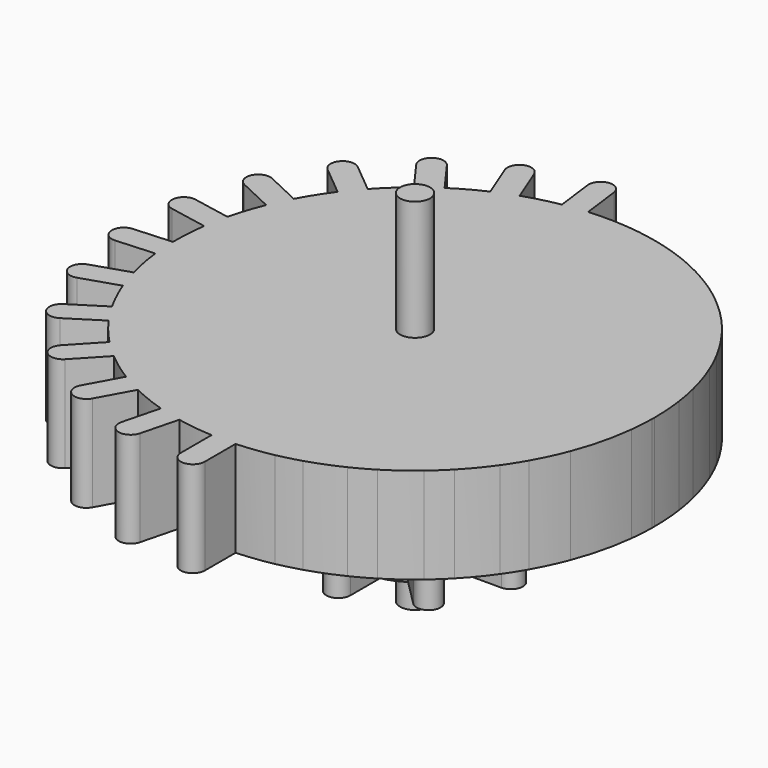
from build123d import *

# Parameters (mm, degrees)
F1_DEPTH      = 10.16
F3_DEPTH      = 10.16
F4_R          = 1.5875
F5_DEPTH      = 12.7
F5_DEPTH_BACK = 25.4


# Not quite as in the source:
# - a feature names something its author has since deleted; it is built from what else it names


with BuildPart() as f1:
    # F0 (on Top) → F1 (new body)
    with BuildSketch(Plane.XY):
        with BuildLine():
            ThreePointArc((6.2217039467, -1.27), (6.3178445716, -0.6382319087), (6.35, 0))
            ThreePointArc((6.35, 0), (6.3178445716, 0.6382319087), (6.2217039467, 1.27))
            ThreePointArc((6.2217039467, 1.27), (5.8666350314, 2.4300397955), (5.2974346633, 3.5013834391))
            ThreePointArc((5.2974346633, 3.5013834391), (4.4901280605, 4.4901280605), (3.5013834391, 5.2974346633))
            ThreePointArc((3.5013834391, 5.2974346633), (2.4300397955, 5.8666350314), (1.27, 6.2217039467))
            ThreePointArc((1.27, 6.2217039467), (0, 6.35), (-1.27, 6.2217039467))
            ThreePointArc((-1.27, 6.2217039467), (-2.4300397955, 5.8666350314), (-3.5013834391, 5.2974346633))
            ThreePointArc((-3.5013834391, 5.2974346633), (-4.4901280605, 4.4901280605), (-5.2974346633, 3.5013834391))
            ThreePointArc((-5.2974346633, 3.5013834391), (-5.8666350314, 2.4300397955), (-6.2217039467, 1.27))
            ThreePointArc((-6.2217039467, 1.27), (-6.35, 0), (-6.2217039467, -1.27))
            ThreePointArc((-6.2217039467, -1.27), (-5.8666350314, -2.4300397955), (-5.2974346633, -3.5013834391))
            ThreePointArc((-5.2974346633, -3.5013834391), (-4.4901280605, -4.4901280605), (-3.5013834391, -5.2974346633))
            ThreePointArc((-3.5013834391, -5.2974346633), (-2.4300397955, -5.8666350314), (-1.27, -6.2217039467))
            ThreePointArc((-1.27, -6.2217039467), (0, -6.35), (1.27, -6.2217039467))
            ThreePointArc((1.27, -6.2217039467), (2.4300397955, -5.8666350314), (3.5013834391, -5.2974346633))
            ThreePointArc((3.5013834391, -5.2974346633), (4.4901280605, -4.4901280605), (5.2974346633, -3.5013834391))
            ThreePointArc((5.2974346633, -3.5013834391), (5.8666350314, -2.4300397955), (6.2217039467, -1.27))
        make_face()
        with BuildLine():
            ThreePointArc((6.2217039467, 1.27), (6.3178445716, 0.6382319087), (6.35, 0))
            ThreePointArc((6.35, 0), (6.3178445716, -0.6382319087), (6.2217039467, -1.27))
            Line((6.2217039467, -1.27), (10.16, -1.27))
            ThreePointArc((10.16, -1.27), (11.43, 0), (10.16, 1.27))
            Line((10.16, 1.27), (6.2217039467, 1.27))
        make_face()
        with BuildLine():
            ThreePointArc((3.5013834391, 5.2974346633), (4.4901280605, 4.4901280605), (5.2974346633, 3.5013834391))
            Line((5.2974346633, 3.5013834391), (8.082230509, 6.2861792847))
            ThreePointArc((8.082230509, 6.2861792847), (8.082230509, 8.082230509), (6.2861792847, 8.082230509))
            Line((6.2861792847, 8.082230509), (3.5013834391, 5.2974346633))
        make_face()
        with BuildLine():
            Line((8.082230509, -6.2861792847), (5.2974346633, -3.5013834391))
            ThreePointArc((5.2974346633, -3.5013834391), (4.4901280605, -4.4901280605), (3.5013834391, -5.2974346633))
            Line((3.5013834391, -5.2974346633), (6.2861792847, -8.082230509))
            ThreePointArc((6.2861792847, -8.082230509), (8.082230509, -8.082230509), (8.082230509, -6.2861792847))
        make_face()
        with BuildLine():
            ThreePointArc((-1.27, 6.2217039467), (0, 6.35), (1.27, 6.2217039467))
            Line((1.27, 6.2217039467), (1.27, 10.16))
            Line((1.27, 10.16), (0, 10.16))
            Line((0, 10.16), (-1.27, 10.16))
            Line((-1.27, 10.16), (-1.27, 6.2217039467))
        make_face()
        with BuildLine():
            Line((1.27, -10.16), (1.27, -6.2217039467))
            ThreePointArc((1.27, -6.2217039467), (0, -6.35), (-1.27, -6.2217039467))
            Line((-1.27, -6.2217039467), (-1.27, -10.16))
            ThreePointArc((-1.27, -10.16), (0, -11.43), (1.27, -10.16))
        make_face()
        with BuildLine():
            Line((0, 10.16), (1.27, 10.16))
            ThreePointArc((1.27, 10.16), (0, 11.43), (-1.27, 10.16))
            Line((-1.27, 10.16), (0, 10.16))
        make_face()
        with BuildLine():
            ThreePointArc((-5.2974346633, 3.5013834391), (-4.4901280605, 4.4901280605), (-3.5013834391, 5.2974346633))
            Line((-3.5013834391, 5.2974346633), (-6.2861792847, 8.082230509))
            ThreePointArc((-6.2861792847, 8.082230509), (-8.082230509, 8.082230509), (-8.082230509, 6.2861792847))
            Line((-8.082230509, 6.2861792847), (-5.2974346633, 3.5013834391))
        make_face()
        with BuildLine():
            Line((-6.2861792847, -8.082230509), (-3.5013834391, -5.2974346633))
            ThreePointArc((-3.5013834391, -5.2974346633), (-4.4901280605, -4.4901280605), (-5.2974346633, -3.5013834391))
            Line((-5.2974346633, -3.5013834391), (-8.082230509, -6.2861792847))
            ThreePointArc((-8.082230509, -6.2861792847), (-8.082230509, -8.082230509), (-6.2861792847, -8.082230509))
        make_face()
        with BuildLine():
            ThreePointArc((-6.2217039467, -1.27), (-6.35, 0), (-6.2217039467, 1.27))
            Line((-6.2217039467, 1.27), (-10.16, 1.27))
            ThreePointArc((-10.16, 1.27), (-11.43, 0), (-10.16, -1.27))
            Line((-10.16, -1.27), (-6.2217039467, -1.27))
        make_face()
    extrude(amount=F1_DEPTH)

    # F2 (on face) → F3 (join)
    with BuildSketch(Plane.XY.offset(10.16)):
        with BuildLine():
            ThreePointArc((25.3979156839, -0.3253904044), (25.3994789156, -0.16269854), (25.4, 0))
            ThreePointArc((25.4, 0), (25.3391429201, 1.7572239685), (25.1568633012, 3.5060275023))
            ThreePointArc((25.1568633012, 3.5060275023), (24.9500961685, 4.7594853905), (24.6809147621, 6.0010371192))
            ThreePointArc((24.6809147621, 6.0010371192), (24.1568355139, 7.8490316571), (23.4946005964, 9.652136697))
            ThreePointArc((23.4946005964, 9.652136697), (22.9826071326, 10.8147940058), (22.4131211958, 11.9503974102))
            ThreePointArc((22.4131211958, 11.9503974102), (21.4459293078, 13.6100005925), (20.356085729, 15.1917666449))
            ThreePointArc((20.356085729, 15.1917666449), (19.5710363665, 16.1905693396), (18.7370287951, 17.1488702815))
            ThreePointArc((18.7370287951, 17.1488702815), (17.3874964906, 18.5158031365), (15.9385231309, 19.7768420231))
            ThreePointArc((15.9385231309, 19.7768420231), (14.9297454082, 20.5490316571), (13.8836199651, 21.2698165639))
            ThreePointArc((13.8836199651, 21.2698165639), (12.2365433222, 22.2581896731), (10.5194845066, 23.1192656829))
            ThreePointArc((10.5194845066, 23.1192656829), (9.3503636382, 23.6163227416), (8.1578522324, 24.0543020467))
            ThreePointArc((8.1578522324, 24.0543020467), (6.316723134, 24.6020122927), (4.4394679828, 25.0090208531))
            ThreePointArc((4.4394679828, 25.0090208531), (3.1834641325, 25.1997134134), (1.9194966415, 25.3273672663))
            ThreePointArc((1.9194966415, 25.3273672663), (0, 25.4), (-1.9194966415, 25.3273672663))
            ThreePointArc((-1.9194966415, 25.3273672663), (-3.1834641325, 25.1997134134), (-4.4394679828, 25.0090208531))
            ThreePointArc((-4.4394679828, 25.0090208531), (-6.316723134, 24.6020122927), (-8.1578522324, 24.0543020467))
            ThreePointArc((-8.1578522324, 24.0543020467), (-9.3503636382, 23.6163227416), (-10.5194845066, 23.1192656829))
            ThreePointArc((-10.5194845066, 23.1192656829), (-12.2365433222, 22.2581896731), (-13.8836199651, 21.2698165639))
            ThreePointArc((-13.8836199651, 21.2698165639), (-14.9297454082, 20.5490316571), (-15.9385231309, 19.7768420231))
            ThreePointArc((-15.9385231309, 19.7768420231), (-17.3874964906, 18.5158031365), (-18.7370287951, 17.1488702815))
            ThreePointArc((-18.7370287951, 17.1488702815), (-19.5710363665, 16.1905693396), (-20.356085729, 15.1917666449))
            ThreePointArc((-20.356085729, 15.1917666449), (-21.4459293078, 13.6100005925), (-22.4131211958, 11.9503974102))
            ThreePointArc((-22.4131211958, 11.9503974102), (-22.9826071326, 10.8147940058), (-23.4946005964, 9.652136697))
            ThreePointArc((-23.4946005964, 9.652136697), (-24.1568355139, 7.8490316571), (-24.6809147621, 6.0010371192))
            ThreePointArc((-24.6809147621, 6.0010371192), (-24.9500961685, 4.7594853905), (-25.1568633012, 3.5060275023))
            ThreePointArc((-25.1568633012, 3.5060275023), (-25.3498789021, 1.594879196), (-25.3979156839, -0.3253904044))
            ThreePointArc((-25.3979156839, -0.3253904044), (-25.3498789021, -1.594879196), (-25.2384277643, -2.8603782946))
            ThreePointArc((-25.2384277643, -2.8603782946), (-24.9500961685, -4.7594853905), (-24.5190721562, -6.6313724521))
            ThreePointArc((-24.5190721562, -6.6313724521), (-24.1568355139, -7.8490316571), (-23.7341689905, -9.0470560035))
            ThreePointArc((-23.7341689905, -9.0470560035), (-22.9826071326, -10.8147940058), (-22.0996051501, -12.5206809802))
            ThreePointArc((-22.0996051501, -12.5206809802), (-21.4459293078, -13.6100005925), (-20.7386050909, -14.665273911))
            ThreePointArc((-20.7386050909, -14.665273911), (-19.5710363665, -16.1905693396), (-18.2915386758, -17.6232690745))
            ThreePointArc((-18.2915386758, -17.6232690745), (-17.3874964906, -18.5158031365), (-16.4399583622, -19.3620187235))
            ThreePointArc((-16.4399583622, -19.3620187235), (-14.9297454082, -20.5490316571), (-13.3341475549, -21.6185223589))
            ThreePointArc((-13.3341475549, -21.6185223589), (-12.2365433222, -22.2581896731), (-11.1083285876, -22.8421766912))
            ThreePointArc((-11.1083285876, -22.8421766912), (-9.3503636382, -23.6163227416), (-7.5389229036, -24.2554043762))
            ThreePointArc((-7.5389229036, -24.2554043762), (-6.316723134, -24.6020122927), (-5.0787216743, -24.8870766896))
            ThreePointArc((-5.0787216743, -24.8870766896), (-3.1834641325, -25.1997134134), (-1.27, -25.3682301314))
            ThreePointArc((-1.27, -25.3682301314), (0, -25.4), (1.27, -25.3682301314))
            ThreePointArc((1.27, -25.3682301314), (3.1834641325, -25.1997134134), (5.0787216743, -24.8870766896))
            ThreePointArc((5.0787216743, -24.8870766896), (6.316723134, -24.6020122927), (7.5389229036, -24.2554043762))
            ThreePointArc((7.5389229036, -24.2554043762), (9.3503636382, -23.6163227416), (11.1083285876, -22.8421766912))
            ThreePointArc((11.1083285876, -22.8421766912), (12.2365433222, -22.2581896731), (13.3341475549, -21.6185223589))
            ThreePointArc((13.3341475549, -21.6185223589), (14.9297454082, -20.5490316571), (16.4399583622, -19.3620187235))
            ThreePointArc((16.4399583622, -19.3620187235), (17.3874964906, -18.5158031365), (18.2915386758, -17.6232690745))
            ThreePointArc((18.2915386758, -17.6232690745), (19.5710363665, -16.1905693396), (20.7386050909, -14.665273911))
            ThreePointArc((20.7386050909, -14.665273911), (21.4459293078, -13.6100005925), (22.0996051501, -12.5206809802))
            ThreePointArc((22.0996051501, -12.5206809802), (22.9826071326, -10.8147940058), (23.7341689905, -9.0470560035))
            ThreePointArc((23.7341689905, -9.0470560035), (24.1568355139, -7.8490316571), (24.5190721562, -6.6313724521))
            ThreePointArc((24.5190721562, -6.6313724521), (24.9500961685, -4.7594853905), (25.2384277643, -2.8603782946))
            ThreePointArc((25.2384277643, -2.8603782946), (25.3498789021, -1.594879196), (25.3979156839, -0.3253904044))
        make_face()
        with BuildLine():
            ThreePointArc((5.2974346633, 3.5013834391), (5.8666350314, 2.4300397955), (6.2217039467, 1.27))
            Line((6.2217039467, 1.27), (10.16, 1.27))
            ThreePointArc((10.16, 1.27), (11.43, 0), (10.16, -1.27))
            Line((10.16, -1.27), (6.2217039467, -1.27))
            ThreePointArc((6.2217039467, -1.27), (5.8666350314, -2.4300397955), (5.2974346633, -3.5013834391))
            Line((5.2974346633, -3.5013834391), (8.082230509, -6.2861792847))
            ThreePointArc((8.082230509, -6.2861792847), (8.082230509, -8.082230509), (6.2861792847, -8.082230509))
            Line((6.2861792847, -8.082230509), (3.5013834391, -5.2974346633))
            ThreePointArc((3.5013834391, -5.2974346633), (2.4300397955, -5.8666350314), (1.27, -6.2217039467))
            Line((1.27, -6.2217039467), (1.27, -10.16))
            ThreePointArc((1.27, -10.16), (0, -11.43), (-1.27, -10.16))
            Line((-1.27, -10.16), (-1.27, -6.2217039467))
            ThreePointArc((-1.27, -6.2217039467), (-2.4300397955, -5.8666350314), (-3.5013834391, -5.2974346633))
            Line((-3.5013834391, -5.2974346633), (-6.2861792847, -8.082230509))
            ThreePointArc((-6.2861792847, -8.082230509), (-8.082230509, -8.082230509), (-8.082230509, -6.2861792847))
            Line((-8.082230509, -6.2861792847), (-5.2974346633, -3.5013834391))
            ThreePointArc((-5.2974346633, -3.5013834391), (-5.8666350314, -2.4300397955), (-6.2217039467, -1.27))
            Line((-6.2217039467, -1.27), (-10.16, -1.27))
            ThreePointArc((-10.16, -1.27), (-11.43, 0), (-10.16, 1.27))
            Line((-10.16, 1.27), (-6.2217039467, 1.27))
            ThreePointArc((-6.2217039467, 1.27), (-5.8666350314, 2.4300397955), (-5.2974346633, 3.5013834391))
            Line((-5.2974346633, 3.5013834391), (-8.082230509, 6.2861792847))
            ThreePointArc((-8.082230509, 6.2861792847), (-8.082230509, 8.082230509), (-6.2861792847, 8.082230509))
            Line((-6.2861792847, 8.082230509), (-3.5013834391, 5.2974346633))
            ThreePointArc((-3.5013834391, 5.2974346633), (-2.4300397955, 5.8666350314), (-1.27, 6.2217039467))
            Line((-1.27, 6.2217039467), (-1.27, 10.16))
            ThreePointArc((-1.27, 10.16), (0, 11.43), (1.27, 10.16))
            Line((1.27, 10.16), (1.27, 6.2217039467))
            ThreePointArc((1.27, 6.2217039467), (2.4300397955, 5.8666350314), (3.5013834391, 5.2974346633))
            Line((3.5013834391, 5.2974346633), (6.2861792847, 8.082230509))
            ThreePointArc((6.2861792847, 8.082230509), (8.082230509, 8.082230509), (8.082230509, 6.2861792847))
            Line((8.082230509, 6.2861792847), (5.2974346633, 3.5013834391))
        make_face(mode=Mode.SUBTRACT)
        with BuildLine():
            Line((10.16, 1.27), (6.2217039467, 1.27))
            ThreePointArc((6.2217039467, 1.27), (5.8666350314, 2.4300397955), (5.2974346633, 3.5013834391))
            Line((5.2974346633, 3.5013834391), (8.082230509, 6.2861792847))
            ThreePointArc((8.082230509, 6.2861792847), (8.082230509, 8.082230509), (6.2861792847, 8.082230509))
            Line((6.2861792847, 8.082230509), (3.5013834391, 5.2974346633))
            ThreePointArc((3.5013834391, 5.2974346633), (2.4300397955, 5.8666350314), (1.27, 6.2217039467))
            Line((1.27, 6.2217039467), (1.27, 10.16))
            ThreePointArc((1.27, 10.16), (0, 11.43), (-1.27, 10.16))
            Line((-1.27, 10.16), (-1.27, 6.2217039467))
            ThreePointArc((-1.27, 6.2217039467), (-2.4300397955, 5.8666350314), (-3.5013834391, 5.2974346633))
            Line((-3.5013834391, 5.2974346633), (-6.2861792847, 8.082230509))
            ThreePointArc((-6.2861792847, 8.082230509), (-8.082230509, 8.082230509), (-8.082230509, 6.2861792847))
            Line((-8.082230509, 6.2861792847), (-5.2974346633, 3.5013834391))
            ThreePointArc((-5.2974346633, 3.5013834391), (-5.8666350314, 2.4300397955), (-6.2217039467, 1.27))
            Line((-6.2217039467, 1.27), (-10.16, 1.27))
            ThreePointArc((-10.16, 1.27), (-11.43, 0), (-10.16, -1.27))
            Line((-10.16, -1.27), (-6.2217039467, -1.27))
            ThreePointArc((-6.2217039467, -1.27), (-5.8666350314, -2.4300397955), (-5.2974346633, -3.5013834391))
            Line((-5.2974346633, -3.5013834391), (-8.082230509, -6.2861792847))
            ThreePointArc((-8.082230509, -6.2861792847), (-8.082230509, -8.082230509), (-6.2861792847, -8.082230509))
            Line((-6.2861792847, -8.082230509), (-3.5013834391, -5.2974346633))
            ThreePointArc((-3.5013834391, -5.2974346633), (-2.4300397955, -5.8666350314), (-1.27, -6.2217039467))
            Line((-1.27, -6.2217039467), (-1.27, -10.16))
            ThreePointArc((-1.27, -10.16), (0, -11.43), (1.27, -10.16))
            Line((1.27, -10.16), (1.27, -6.2217039467))
            ThreePointArc((1.27, -6.2217039467), (2.4300397955, -5.8666350314), (3.5013834391, -5.2974346633))
            Line((3.5013834391, -5.2974346633), (6.2861792847, -8.082230509))
            ThreePointArc((6.2861792847, -8.082230509), (8.082230509, -8.082230509), (8.082230509, -6.2861792847))
            Line((8.082230509, -6.2861792847), (5.2974346633, -3.5013834391))
            ThreePointArc((5.2974346633, -3.5013834391), (5.8666350314, -2.4300397955), (6.2217039467, -1.27))
            Line((6.2217039467, -1.27), (10.16, -1.27))
            ThreePointArc((10.16, -1.27), (11.43, 0), (10.16, 1.27))
        make_face()
        with BuildLine():
            ThreePointArc((-23.4946005964, 9.652136697), (-22.9826071326, 10.8147940058), (-22.4131211958, 11.9503974102))
            Line((-22.4131211958, 11.9503974102), (-26.0993233564, 13.6849924804))
            ThreePointArc((-26.0993233564, 13.6849924804), (-27.7891934134, 13.076601824), (-27.180802757, 11.3867317671))
            Line((-27.180802757, 11.3867317671), (-23.4946005964, 9.652136697))
        make_face()
        with BuildLine():
            ThreePointArc((-20.356085729, 15.1917666449), (-19.5710363665, 16.1905693396), (-18.7370287951, 17.1488702815))
            Line((-18.7370287951, 17.1488702815), (-21.8760458841, 19.7456910573))
            ThreePointArc((-21.8760458841, 19.7456910573), (-23.6641261694, 19.5766677059), (-23.4951028181, 17.7885874206))
            Line((-23.4951028181, 17.7885874206), (-20.356085729, 15.1917666449))
        make_face()
        with BuildLine():
            ThreePointArc((-15.9385231309, 19.7768420231), (-14.9297454082, 20.5490316571), (-13.8836199651, 21.2698165639))
            Line((-13.8836199651, 21.2698165639), (-16.2782159944, 24.5656952454))
            ThreePointArc((-16.2782159944, 24.5656952454), (-18.0521548477, 24.8466595579), (-18.3331191601, 23.0727207046))
            Line((-18.3331191601, 23.0727207046), (-15.9385231309, 19.7768420231))
        make_face()
        with BuildLine():
            ThreePointArc((-10.5194845066, 23.1192656829), (-9.3503636382, 23.6163227416), (-8.1578522324, 24.0543020467))
            Line((-8.1578522324, 24.0543020467), (-9.6575659267, 27.842146455))
            ThreePointArc((-9.6575659267, 27.842146455), (-11.3059002457, 28.5554444102), (-12.0191982008, 26.9071100912))
            Line((-12.0191982008, 26.9071100912), (-10.5194845066, 23.1192656829))
        make_face()
        with BuildLine():
            ThreePointArc((-25.1568633012, 3.5060275023), (-24.9500961685, 4.7594853905), (-24.6809147621, 6.0010371192))
            Line((-24.6809147621, 6.0010371192), (-28.6826843557, 6.7644154961))
            ThreePointArc((-28.6826843557, 6.7644154961), (-30.1681634337, 5.7548849572), (-29.1586328948, 4.2694058792))
            Line((-29.1586328948, 4.2694058792), (-25.1568633012, 3.5060275023))
        make_face()
        with BuildLine():
            ThreePointArc((-25.2384277643, -2.8603782946), (-25.3498789021, -1.594879196), (-25.3979156839, -0.3253904044))
            Line((-25.3979156839, -0.3253904044), (-29.4638068094, -0.5811945916))
            ThreePointArc((-29.4638068094, -0.5811945916), (-30.6515567947, -1.9284324965), (-29.3043188898, -3.1161824818))
            Line((-29.3043188898, -3.1161824818), (-25.2384277643, -2.8603782946))
        make_face()
        with BuildLine():
            Line((-27.6087067552, -10.3059696371), (-23.7341689905, -9.0470560035))
            ThreePointArc((-23.7341689905, -9.0470560035), (-24.1568355139, -7.8490316571), (-24.5190721562, -6.6313724521))
            Line((-24.5190721562, -6.6313724521), (-28.3936099209, -7.8902860857))
            ThreePointArc((-28.3936099209, -7.8902860857), (-29.2090001137, -9.4905794442), (-27.6087067552, -10.3059696371))
        make_face()
        with BuildLine():
            Line((-24.1783380374, -16.8481948173), (-20.7386050909, -14.665273911))
            ThreePointArc((-20.7386050909, -14.665273911), (-21.4459293078, -13.6100005925), (-22.0996051501, -12.5206809802))
            Line((-22.0996051501, -12.5206809802), (-25.5393380967, -14.7036018865))
            ThreePointArc((-25.5393380967, -14.7036018865), (-25.9311345324, -16.4563983815), (-24.1783380374, -16.8481948173))
        make_face()
        with BuildLine():
            Line((-19.2287554191, -22.3317859538), (-16.4399583622, -19.3620187235))
            ThreePointArc((-16.4399583622, -19.3620187235), (-17.3874964906, -18.5158031365), (-18.2915386758, -17.6232690745))
            Line((-18.2915386758, -17.6232690745), (-21.0803357327, -20.5930363047))
            ThreePointArc((-21.0803357327, -20.5930363047), (-21.0239204004, -22.3882012861), (-19.2287554191, -22.3317859538))
        make_face()
        with BuildLine():
            Line((-13.0709593794, -26.4121888482), (-11.1083285876, -22.8421766912))
            ThreePointArc((-11.1083285876, -22.8421766912), (-12.2365433222, -22.2581896731), (-13.3341475549, -21.6185223589))
            Line((-13.3341475549, -21.6185223589), (-15.2967783467, -25.188534516))
            ThreePointArc((-15.2967783467, -25.188534516), (-14.7956960291, -26.9132711658), (-13.0709593794, -26.4121888482))
        make_face()
        with BuildLine():
            Line((-6.0918668902, -28.8330167802), (-5.0787216743, -24.8870766896))
            ThreePointArc((-5.0787216743, -24.8870766896), (-6.316723134, -24.6020122927), (-7.5389229036, -24.2554043762))
            Line((-7.5389229036, -24.2554043762), (-8.5520681195, -28.2013444668))
            ThreePointArc((-8.5520681195, -28.2013444668), (-7.6378036615, -29.7472812381), (-6.0918668902, -28.8330167802))
        make_face()
        with BuildLine():
            Line((1.27, -29.4421602273), (1.27, -25.3682301314))
            ThreePointArc((1.27, -25.3682301314), (0, -25.4), (-1.27, -25.3682301314))
            Line((-1.27, -25.3682301314), (-1.27, -29.4421602273))
            ThreePointArc((-1.27, -29.4421602273), (0, -30.7121602273), (1.27, -29.4421602273))
        make_face()
        with BuildLine():
            ThreePointArc((-4.4394679828, 25.0090208531), (-3.1834641325, 25.1997134134), (-1.9194966415, 25.3273672663))
            Line((-1.9194966415, 25.3273672663), (-2.4300954737, 29.3691732066))
            Line((-2.4300954737, 29.3691732066), (-3.6900811444, 29.21))
            Line((-3.6900811444, 29.21), (-4.9500668151, 29.0508267934))
            Line((-4.9500668151, 29.0508267934), (-4.4394679828, 25.0090208531))
        make_face()
        with BuildLine():
            Line((-3.6900811444, 29.21), (-2.4300954737, 29.3691732066))
            ThreePointArc((-2.4300954737, 29.3691732066), (-3.849254351, 30.4699856707), (-4.9500668151, 29.0508267934))
            Line((-4.9500668151, 29.0508267934), (-3.6900811444, 29.21))
        make_face()
    extrude(amount=F3_DEPTH)

    # F4 (on face) → F5 (join, two sides)
    with BuildSketch(Plane.XY.offset(20.32)) as f5_sk:
        Circle(F4_R)
    extrude(amount=F5_DEPTH)
    extrude(f5_sk.sketch, amount=-F5_DEPTH_BACK)


solid = f1.part
